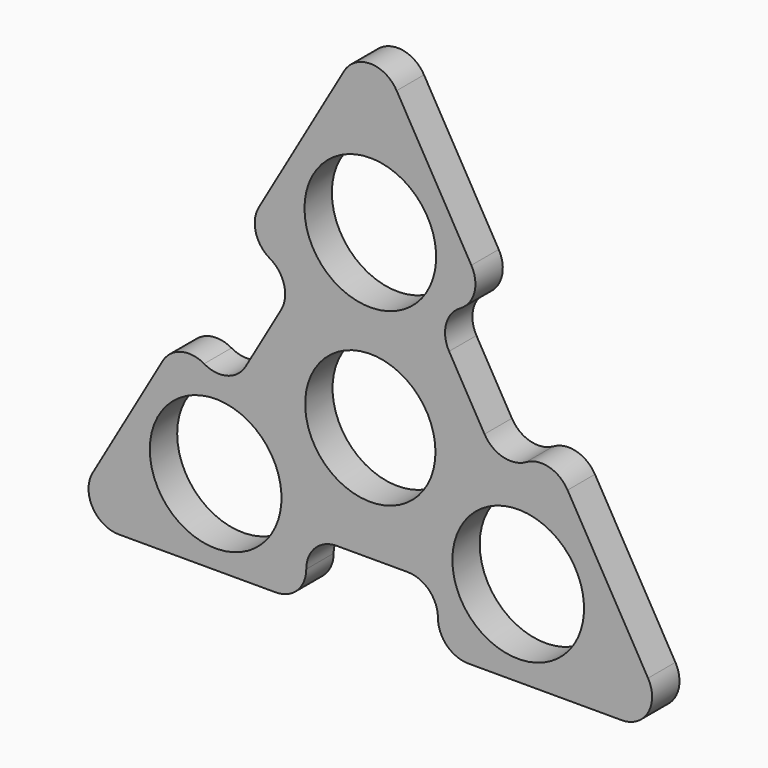
from build123d import *

# Parameters (mm, degrees)
F1_DEPTH  = 5.715
F2_R      = 10.8839
F3_DEPTH  = 25.4
F4_W      = 5.715
F4_H      = 21.9964
F5_DEPTH  = 10.16
F6_R      = 5.07999
F7_R      = 5.08
F8_W      = 5.715
F8_H      = 21.9964
F9_DEPTH  = 10.16
F10_R     = 5.07999
F11_W     = 21.9964
F11_H     = 5.715
F12_DEPTH = 10.16
F13_R     = 5.07999
F14_R     = 10.9982
F15_DEPTH = 25.4


# Not quite as in the source:
# - a fillet or chamfer is up to 0.001 mm smaller than in the source, because OpenCascade refuses the exact size


with BuildPart() as f1:
    # F0 (on Front) → F1 (new body)
    with BuildSketch(Plane.XZ):
        Polygon((-50.8, -29.3293936748), (50.8, -29.3293936748), (0, 58.6587873497), align=None)
    extrude(amount=F1_DEPTH)

    # F2 (on face) → F3 (cut)
    with BuildSketch(Plane.XZ.offset(5.715)):
        Circle(F2_R)
    extrude(amount=-F3_DEPTH, mode=Mode.SUBTRACT)

    # F4 (on face) → F5 (cut)
    with BuildSketch(Plane(origin=(25.4, 0, 14.6646968374), x_dir=(0, 1, 0), z_dir=(0.8660254038, 0, 0.5))):
        with Locations((-2.8575, 0.9615815512)):
            Rectangle(F4_W, F4_H)
    extrude(amount=-F5_DEPTH, mode=Mode.SUBTRACT)

    # F6 (radius 5.08 in the source; OpenCascade refuses exactly that, so slightly less here)
    f6_edges = [f1.edges().sort_by_distance(p)[0] for p in [
        (21.619491, -2.8575, 0.89273),
        (10.621291, -2.8575, 19.942171),
        (30.418309, -2.8575, 5.97273),
        (19.420109, -2.8575, 25.022171),
    ]]
    fillet(f6_edges, radius=F6_R)

    # F7
    f7_edges = [f1.edges().sort_by_distance(p)[0] for p in [
        (50.8, -2.8575, -29.329394),
        (-50.8, -2.8575, -29.329394),
        (0, -2.8575, 58.658787),
    ]]
    fillet(f7_edges, radius=F7_R)

    # F8 (on face) → F9 (cut)
    with BuildSketch(Plane(origin=(-25.4, 0, 14.6646968374), x_dir=(0, -1, 0), z_dir=(-0.8660254038, 0, 0.5))):
        with Locations((2.8575, -2.5338024565)):
            Rectangle(F8_W, F8_H)
    extrude(amount=-F9_DEPTH, mode=Mode.SUBTRACT)

    # F10 (radius 5.08 in the source; OpenCascade refuses exactly that, so slightly less here)
    f10_edges = [f1.edges().sort_by_distance(p)[0] for p in [
        (-21.167801, -2.8575, 21.99508),
        (-12.368983, -2.8575, 16.91508),
        (-32.166001, -2.8575, 2.945639),
        (-23.367183, -2.8575, -2.134361),
    ]]
    fillet(f10_edges, radius=F10_R)

    # F11 (on face) → F12 (cut)
    with BuildSketch(Plane(origin=(0, 0, -29.3293936748), x_dir=(1, 0, 0), z_dir=(0, 0, -1))):
        with Locations((0.2968947671, 2.8575)):
            Rectangle(F11_W, F11_H)
    extrude(amount=-F12_DEPTH, mode=Mode.SUBTRACT)

    # F13 (radius 5.08 in the source; OpenCascade refuses exactly that, so slightly less here)
    f13_edges = [f1.edges().sort_by_distance(p)[0] for p in [
        (11.295095, -2.8575, -29.329394),
        (11.295095, -2.8575, -19.169394),
        (-10.701305, -2.8575, -29.329394),
        (-10.701305, -2.8575, -19.169394),
    ]]
    fillet(f13_edges, radius=F13_R)

    # F14 (on face) → F15 (cut)
    with BuildSketch(Plane(origin=(0, 0, 0), x_dir=(-1, 0, 0), z_dir=(0, 1, 0))):
        with Locations((0, 28.7260549402)):
            Circle(F14_R)
        with Locations((25.8424041398, -15.1333886554)):
            Circle(F14_R)
        with Locations((-24.7085423876, -14.9420522576)):
            Circle(F14_R)
    extrude(amount=-F15_DEPTH, mode=Mode.SUBTRACT)


solid = f1.part
